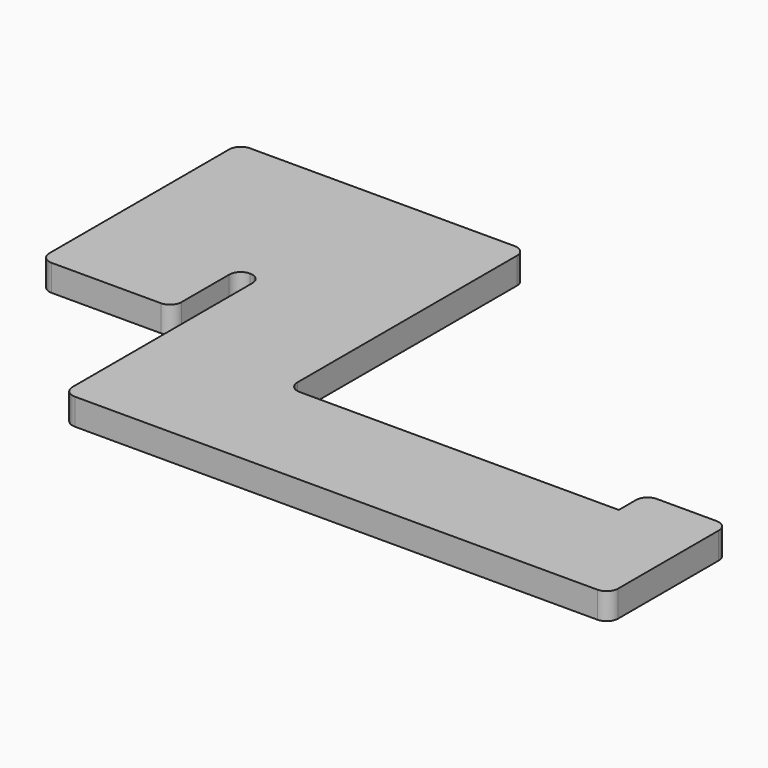
from build123d import *

# Parameters (mm, degrees)
F1_DEPTH = 2.032
F2_R     = 0.88899


# Not quite as in the source:
# - a fillet or chamfer is up to 0.001 mm smaller than in the source, because OpenCascade refuses the exact size


with BuildPart() as f1:
    # F0 (on Top) → F1 (new body)
    with BuildSketch(Plane.XY):
        Polygon((11.938, 12.7), (-10.16, 12.7), (-10.16, -6.35), (0, -6.35), (0, 0), (1.778, 0), (1.778, -19.05), (43.688, -19.05), (43.688, -7.62), (37.338, -7.62), (37.338, -10.16), (11.938, -10.16), align=None)
    extrude(amount=F1_DEPTH)

    # F2 (radius 0.889 in the source; OpenCascade refuses exactly that, so slightly less here)
    f2_edges = [f1.edges().sort_by_distance(p)[0] for p in [
        (-10.16, -6.35, 1.016),
        (0, -6.35, 1.016),
        (0, 0, 1.016),
        (1.778, 0, 1.016),
        (1.778, -19.05, 1.016),
        (-10.16, 12.7, 1.016),
        (37.338, -7.62, 1.016),
        (43.688, -19.05, 1.016),
        (11.938, 12.7, 1.016),
        (11.938, -10.16, 1.016),
        (43.688, -7.62, 1.016),
    ]]
    fillet(f2_edges, radius=F2_R)


solid = f1.part
